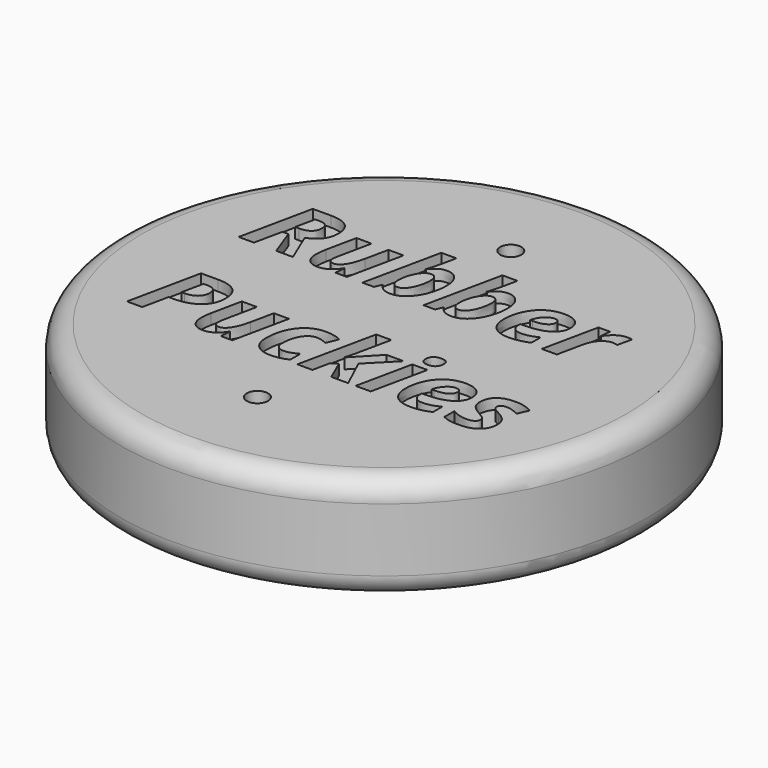
from build123d import *

# Parameters (mm, degrees)
F0_R           = 25
F1_DEPTH       = 10
F2_TEXT_SIZE   = 9.7222222222
F3_DEPTH       = 1
F4_R           = 2
F6_D           = 2
F6_CBORE_D     = 5
F6_CBORE_DEPTH = 2.5


# Not quite as in the source:
# - Text() gives the source's letters only with a copy of the font that has no kerning and outlines rounded to 1/6400 em; it was checked with that copy


with BuildPart() as f1:
    # F0 (on Top) → F1 (new body)
    with BuildSketch(Plane.XY):
        Circle(F0_R)
    extrude(amount=F1_DEPTH)

    # F2 (on face) → F3 (cut)
    with BuildSketch(Plane.XY.offset(10)):
        with Locations((-17.3602830619, 4.1679781862)):
            Text('Rubber', F2_TEXT_SIZE, font='Open Sans', font_style=FontStyle.BOLDITALIC, text_align=(TextAlign.LEFT, TextAlign.BOTTOM))
        with Locations((-17.3602830619, -9.0542440361)):
            Text('Puckies', F2_TEXT_SIZE, font='Open Sans', font_style=FontStyle.BOLDITALIC, text_align=(TextAlign.LEFT, TextAlign.BOTTOM))
    extrude(amount=-F3_DEPTH, mode=Mode.SUBTRACT)

    # F4
    f4_edges = [f1.edges().sort_by_distance(p)[0] for p in [
        (-25, 0, 10),
        (-25, 0, 0),
    ]]
    fillet(f4_edges, radius=F4_R)

    # F6 (through all)
    with Locations(Plane(origin=(0, 0, 0), x_dir=(1, 0, 0), z_dir=(0, 0, -1))):
        with Locations((0, 15), (0, -15)):
            CounterBoreHole(F6_D / 2, F6_CBORE_D / 2, F6_CBORE_DEPTH)


solid = f1.part
